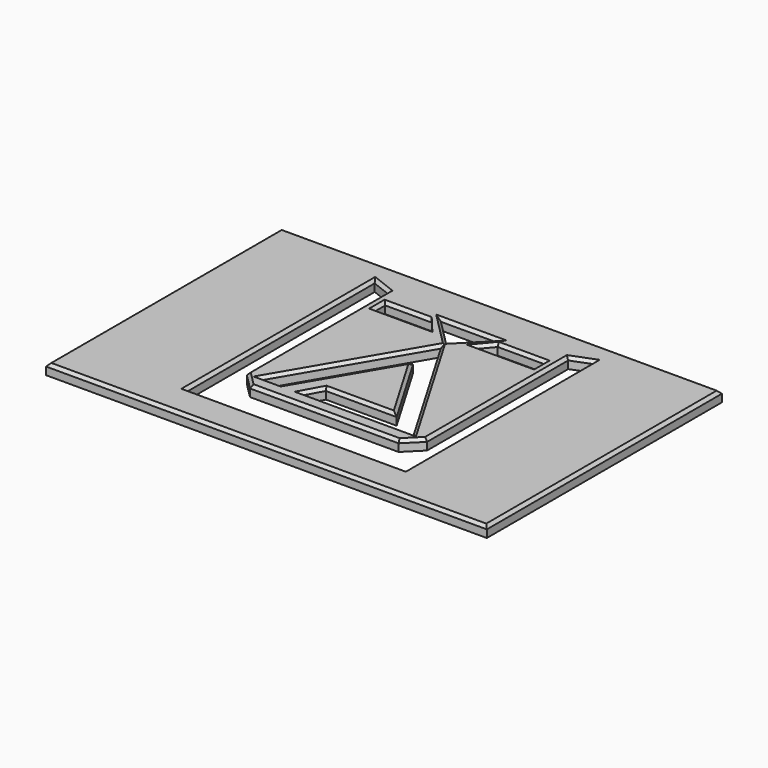
from build123d import *

# Parameters (mm, degrees)
F2_DEPTH      = 0.9
F3_DEPTH      = 5
F4_T1_DEPTH   = 26.285841494
F4_T3_DEPTH   = 38.785841494
F4_T5_DEPTH   = 3.1950298032
F4_T7_DEPTH   = 13.9251834597
F4_T9_DEPTH   = 3.1950298032
F4_T11_DEPTH  = 18.6
F4_T13_DEPTH  = 8.9042054248
F4_T15_DEPTH  = 1.1497265659
F4_T20_DEPTH  = 20.642920747
F4_T25_DEPTH  = 3.035841494
F4_T31_DEPTH  = 16.285841494
F4_T36_DEPTH  = 16.285841494
F4_T41_DEPTH  = 3.035841494
F4_T47_DEPTH  = 20.642920747
F4_T52_DEPTH  = 14.073841494
F4_T58_DEPTH  = 14.073841494
F4_T64_DEPTH  = 10.6487776251
F4_T69_DEPTH  = 7.3005243293
F4_T74_DEPTH  = 3.0018588708
F4_T80_DEPTH  = 10.7389121025
F4_T86_DEPTH  = 3.0133324052
F4_T92_DEPTH  = 5.5681345012
F4_T97_DEPTH  = 4.6046142425
F4_T102_DEPTH = 4.7067640091
F4_T108_DEPTH = 6.1091194569
F4_T114_DEPTH = 4.7067640091
F4_T120_DEPTH = 2.7859223136
F4_T126_DEPTH = 4.6046142425
F4_T131_DEPTH = 5.5681345012
F4_T137_DEPTH = 19.242920747
F4_T141_DEPTH = 21.285841494
F4_T148_DEPTH = 3.035841494
F4_T152_DEPTH = 20.642920747
F4_T159_DEPTH = 16.285841494
F4_T163_DEPTH = 3.035841494
F4_T170_DEPTH = 3.035841494
F4_T174_DEPTH = 16.285841494
F4_T181_DEPTH = 20.642920747
F4_T185_DEPTH = 3.035841494
F4_T192_DEPTH = 19.242920747
F4_T196_DEPTH = 21.285841494
F4_T203_DEPTH = 3.0133324052
F4_T207_DEPTH = 14.073841494
F4_T214_DEPTH = 14.073841494
F4_T218_DEPTH = 14.073841494
F4_T225_DEPTH = 10.7389121025
F4_T229_DEPTH = 14.073841494
F4_T236_DEPTH = 3.0133324052
F4_T240_DEPTH = 10.6487776251
F4_T247_DEPTH = 7.3005243293
F4_T251_DEPTH = 3.0018588708
F4_T258_DEPTH = 3.0018588708
F4_T262_DEPTH = 10.7389121025
F4_T269_DEPTH = 1.7926473129
F4_T273_DEPTH = 6.2110552482
F4_T280_DEPTH = 1.7926473129
F4_T284_DEPTH = 5.2475349895
F4_T291_DEPTH = 4.7067640091
F4_T295_DEPTH = 4.7067640091
F4_T302_DEPTH = 6.1091194569
F4_T306_DEPTH = 4.7067640091
F4_T313_DEPTH = 6.1091194569
F4_T317_DEPTH = 4.7067640091
F4_T324_DEPTH = 2.7859223136
F4_T328_DEPTH = 5.5681345012
F4_T335_DEPTH = 4.6046142425
F4_T339_DEPTH = 2.7859223136
F4_T346_DEPTH = 5.2475349895
F4_T350_DEPTH = 1.7926473129
F4_T357_DEPTH = 6.2110552482
F4_T361_DEPTH = 1.7926473129


# Not quite as in the source:
# - a fillet or chamfer that OpenCascade refuses, or shapes differently, is made with other operations: its cross-section is extruded or revolved along the edge and cut away or added


with BuildPart() as f2:
    # F1 (on Top) → F2 (new body)
    with BuildSketch(Plane.XY):
        Polygon((-18.75, -12), (0, -12), (18.75, -12), (18.75, 13), (-18.75, 13), align=None)
    extrude(amount=F2_DEPTH)

    # F0 (on Top) → F3 (cut)
    with BuildSketch(Plane.XY):
        Polygon((-9.1827595606, 10.9884138033), (-9.1827595606, -9.0115861967), (9.4172404394, -9.0115861967), (9.4172404394, 10.9884138033), (7.7869114222, 10.3523892), (7.7869114222, -4.6476108), (6.4369114222, -5.9976108), (-6.2024305435, -5.9976108), (-7.5524305435, -4.6476108), (-7.5524305435, 10.3523892), align=None)
        Polygon((-2.6888800301, 8.9422948658), (-6.6505735256, 8.9422948658), (-6.6505735256, 7.7925682999), (-1.7253597714, 7.7925682999), align=None)
        Polygon((0.1172404394, 6.394509411), (-6.3555088598, -4.6343826689), (-4.6280179486, -4.6343826689), (0.1170416773, 3.4371092715), (3.9779663485, -3.1304419972), (-2.0367164869, -3.1304419972), (-2.86308087, -4.6343826689), (6.5899897385, -4.6343826689), align=None)
        Polygon((6.8850544043, 8.9422948658), (2.9233609088, 8.9422948658), (1.9598406501, 7.7925682999), (6.8850544043, 7.7925682999), align=None)
        Polygon((2.5288794208, 9.4185657799), (-2.2943985421, 9.4185657799), (0.1172404394, 6.9923118202), align=None)
    extrude(amount=F3_DEPTH, mode=Mode.SUBTRACT)

    # F4: chamfer of 0.25 on 32 edges, made by hand

    # F4_s2 → F4_t1 (cut)
    with BuildSketch(Plane.XZ.offset(-13.642920747)):
        Polygon((-18.75, 0.65), (-18.5, 0.9), (-18.75, 0.9), align=None)
        Polygon((18.5, 0.9), (18.75, 0.65), (18.75, 0.9), align=None)
    extrude(amount=F4_T1_DEPTH, mode=Mode.SUBTRACT)

    # F4_s4 → F4_t3 (cut)
    with BuildSketch(Plane.YZ.offset(-19.392920747)):
        Polygon((12.75, 0.9), (13, 0.65), (13, 0.9), align=None)
        Polygon((-12, 0.65), (-11.75, 0.9), (-12, 0.9), align=None)
    extrude(amount=F4_T3_DEPTH, mode=Mode.SUBTRACT)

    # F4_s6 → F4_t5 (cut)
    with BuildSketch(Plane(origin=(-1.9070234917, 1.9070234917, 0), x_dir=(0, 0, 1), z_dir=(0.7071067812, -0.7071067812, 0))):
        Polygon((0.9, 8.3767319647), (0.65, 8.6267319647), (0.9, 8.6267319647), align=None)
    extrude(amount=F4_T5_DEPTH, mode=Mode.SUBTRACT)

    # F4_s8 → F4_t7 (cut)
    with BuildSketch(Plane.YZ.offset(-6.8453512905)):
        Polygon((-5.7476108, 0.9), (-5.9976108, 0.65), (-5.9976108, 0.9), align=None)
    extrude(amount=F4_T7_DEPTH, mode=Mode.SUBTRACT)

    # F4_s10 → F4_t9 (cut)
    with BuildSketch(Plane(origin=(-0.2349633088, -0.2349633088, 0), x_dir=(0, 0, 1), z_dir=(0.7071067812, 0.7071067812, 0))):
        Polygon((0.9, 8.5425349841), (0.65, 8.7925349841), (0.9, 8.7925349841), align=None)
    extrude(amount=F4_T9_DEPTH, mode=Mode.SUBTRACT)

    # F4_s12 → F4_t11 (cut)
    with BuildSketch(Plane.YZ.offset(-9.1827595606)):
        Polygon((-9.2615861967, 0.9), (-9.0115861967, 0.65), (-9.0115861967, 0.9), align=None)
    extrude(amount=F4_T11_DEPTH, mode=Mode.SUBTRACT)

    # F4_s14 → F4_t13 (cut)
    with BuildSketch(Plane(origin=(2.7151762758, -4.6185981114, 0), x_dir=(0, 0, 1), z_dir=(-0.5067918396, 0.8620684609, 0))):
        Polygon((0.9, 1.5927968692), (0.65, 1.8427968692), (0.9, 1.8427968692), align=None)
    extrude(amount=F4_T13_DEPTH, mode=Mode.SUBTRACT)

    # F4_s16 → F4_t15 (cut)
    with BuildSketch(Plane.XZ.offset(-8.9422948658)):
        Polygon((-6.9005735256, 0.9), (-6.6505735256, 0.65), (-6.6505735256, 0.9), align=None)
        Polygon((7.1350544043, 0.9), (6.8850544043, 0.65), (6.8850544043, 0.9), align=None)
    extrude(amount=F4_T15_DEPTH, mode=Mode.SUBTRACT)


with BuildPart() as f4_tool18:
    # F4_s19 → F4_t20 (new body)
    with BuildSketch(Plane.XZ.offset(9.0115861967)):
        Polygon((-9.4327595606, 0.9), (-9.1827595606, 0.65), (-9.1827595606, 0.9), align=None)
    extrude(amount=-F4_T20_DEPTH)

    split(bisect_by=Plane(origin=(2.5076023076, 6.4277651912, 0), x_dir=(0, 0, 1), z_dir=(-0.3634426304, -0.9316165812, 0)), keep=Keep.TOP)


with BuildPart() as f2_1:
    add(f2.part)

    # F4_t17: cut F4_tool18
    add(f4_tool18.part, mode=Mode.SUBTRACT)


with BuildPart() as f4_tool23:
    # F4_s24 → F4_t25 (new body)
    with BuildSketch(Plane(origin=(-12.2893174966, 4.7943134195, 0), x_dir=(0, 0, 1), z_dir=(0.9316165812, -0.3634426304, 0))):
        Polygon((0.9, -7.149582211), (0.65, -6.899582211), (0.9, -6.899582211), align=None)
    extrude(amount=F4_T25_DEPTH)

    split(bisect_by=Plane.YZ.offset(-7.5524305435), keep=Keep.BOTTOM)

    split(bisect_by=Plane.YZ.offset(-9.1827595606), keep=Keep.TOP)


with BuildPart() as f2_2:
    add(f2_1.part)

    # F4_t22: cut F4_tool23
    add(f4_tool23.part, mode=Mode.SUBTRACT)


with BuildPart() as f4_tool29:
    # F4_s30 → F4_t31 (new body)
    with BuildSketch(Plane.XZ.offset(-10.995309947)):
        Polygon((-7.3024305435, 0.9), (-7.5524305435, 0.65), (-7.5524305435, 0.9), align=None)
    extrude(amount=F4_T31_DEPTH)

    split(bisect_by=Plane(origin=(2.5076023076, 6.4277651912, 0), x_dir=(0, 0, 1), z_dir=(-0.3634426304, -0.9316165812, 0)), keep=Keep.TOP)


with BuildPart() as f2_3:
    add(f2_2.part)

    # F4_t28: cut F4_tool29
    add(f4_tool29.part, mode=Mode.SUBTRACT)


with BuildPart() as f4_tool34:
    # F4_s35 → F4_t36 (new body)
    with BuildSketch(Plane.XZ.offset(5.290531547)):
        Polygon((7.5369114222, 0.9), (7.7869114222, 0.65), (7.7869114222, 0.9), align=None)
    extrude(amount=-F4_T36_DEPTH)

    split(bisect_by=Plane(origin=(-2.4766296004, 6.3483725026, 0), x_dir=(0, 0, 1), z_dir=(0.3634426304, -0.9316165812, 0)), keep=Keep.TOP)


with BuildPart() as f2_4:
    add(f2_3.part)

    # F4_t33: cut F4_tool34
    add(f4_tool34.part, mode=Mode.SUBTRACT)


with BuildPart() as f4_tool39:
    # F4_s40 → F4_t41 (new body)
    with BuildSketch(Plane(origin=(9.6645853944, 3.77035189, 0), x_dir=(0, 0, 1), z_dir=(0.9316165812, 0.3634426304, 0))):
        Polygon((0.9, -7.0643618637), (0.65, -6.8143618637), (0.9, -6.8143618637), align=None)
    extrude(amount=F4_T41_DEPTH)

    split(bisect_by=Plane.YZ.offset(9.4172404394), keep=Keep.BOTTOM)

    split(bisect_by=Plane.YZ.offset(7.7869114222), keep=Keep.TOP)


with BuildPart() as f2_5:
    add(f2_4.part)

    # F4_t38: cut F4_tool39
    add(f4_tool39.part, mode=Mode.SUBTRACT)


with BuildPart() as f4_tool45:
    # F4_s46 → F4_t47 (new body)
    with BuildSketch(Plane.XZ.offset(-11.6313345503)):
        Polygon((9.6672404394, 0.9), (9.4172404394, 0.65), (9.4172404394, 0.9), align=None)
    extrude(amount=F4_T47_DEPTH)

    split(bisect_by=Plane(origin=(-2.4766296004, 6.3483725026, 0), x_dir=(0, 0, 1), z_dir=(0.3634426304, -0.9316165812, 0)), keep=Keep.TOP)


with BuildPart() as f2_6:
    add(f2_5.part)

    # F4_t44: cut F4_tool45
    add(f4_tool45.part, mode=Mode.SUBTRACT)


with BuildPart() as f4_tool50:
    # F4_s51 → F4_t52 (new body)
    with BuildSketch(Plane(origin=(-3.9767285934, -6.7759322138, 0), x_dir=(0, 0, 1), z_dir=(0.5061580622, 0.8624407319, 0))):
        Polygon((0.9, -3.3855195618), (0.65, -3.1355195618), (0.9, -3.1355195618), align=None)
    extrude(amount=F4_T52_DEPTH)

    split(bisect_by=Plane.XZ.offset(4.6343826689), keep=Keep.BOTTOM)

    split(bisect_by=Plane(origin=(2.8786076051, 1.6894267551, 0), x_dir=(0, 0, 1), z_dir=(-0.8624407319, -0.5061580622, 0)), keep=Keep.TOP)


with BuildPart() as f2_7:
    add(f2_6.part)

    # F4_t49: cut F4_tool50
    add(f4_tool50.part, mode=Mode.SUBTRACT)


with BuildPart() as f4_tool56:
    # F4_s57 → F4_t58 (new body)
    with BuildSketch(Plane(origin=(-3.0867866852, 5.2595636956, 0), x_dir=(0, 0, 1), z_dir=(0.5061580622, -0.8624407319, 0))):
        Polygon((0.9, -3.5877454224), (0.65, -3.3377454224), (0.9, -3.3377454224), align=None)
    extrude(amount=F4_T58_DEPTH)

    split(bisect_by=Plane.XZ.offset(4.6343826689), keep=Keep.BOTTOM)

    split(bisect_by=Plane(origin=(-2.7041997858, 1.5870685053, 0), x_dir=(0, 0, 1), z_dir=(0.8624407319, -0.5061580622, 0)), keep=Keep.TOP)


with BuildPart() as f2_8:
    add(f2_7.part)

    # F4_t55: cut F4_tool56
    add(f4_tool56.part, mode=Mode.SUBTRACT)


with BuildPart() as f4_tool62:
    # F4_s63 → F4_t64 (new body)
    with BuildSketch(Plane(origin=(1.8575238649, 3.1597050588, 0), x_dir=(0, 0, 1), z_dir=(-0.5067918396, -0.8620684609, 0))):
        Polygon((0.9, 1.391000992), (0.65, 1.641000992), (0.9, 1.641000992), align=None)
    extrude(amount=F4_T64_DEPTH)

    split(bisect_by=Plane.XZ.offset(4.6343826689), keep=Keep.BOTTOM)


with BuildPart() as f2_9:
    add(f2_8.part)

    # F4_t61: cut F4_tool62
    add(f4_tool62.part, mode=Mode.SUBTRACT)


with BuildPart() as f4_tool67:
    # F4_s68 → F4_t69 (new body)
    with BuildSketch(Plane.YZ.offset(-2.6796372339)):
        Polygon((-2.8804419972, 0.9), (-3.1304419972, 0.65), (-3.1304419972, 0.9), align=None)
    extrude(amount=F4_T69_DEPTH)

    split(bisect_by=Plane(origin=(-0.2432150273, 0.1336384073, 0), x_dir=(0, 0, 1), z_dir=(0.876413428, -0.4815594494, 0)), keep=Keep.TOP)


with BuildPart() as f2_10:
    add(f2_9.part)

    # F4_t66: cut F4_tool67
    add(f4_tool67.part, mode=Mode.SUBTRACT)


with BuildPart() as f4_tool72:
    # F4_s73 → F4_t74 (new body)
    with BuildSketch(Plane(origin=(-2.9294704036, -5.3314854519, 0), x_dir=(0, 0, 1), z_dir=(0.4815594494, 0.876413428, 0))):
        Polygon((0.9, -0.5275117536), (0.65, -0.2775117536), (0.9, -0.2775117536), align=None)
    extrude(amount=F4_T74_DEPTH)

    split(bisect_by=Plane.XZ.offset(3.1304419972), keep=Keep.TOP)

    split(bisect_by=Plane.XZ.offset(4.6343826689), keep=Keep.BOTTOM)


with BuildPart() as f2_11:
    add(f2_10.part)

    # F4_t71: cut F4_tool72
    add(f4_tool72.part, mode=Mode.SUBTRACT)


with BuildPart() as f4_tool78:
    # F4_s79 → F4_t80 (new body)
    with BuildSketch(Plane.YZ.offset(7.2329104855)):
        Polygon((-4.8843826689, 0.9), (-4.6343826689, 0.65), (-4.6343826689, 0.9), align=None)
    extrude(amount=-F4_T80_DEPTH)

    split(bisect_by=Plane(origin=(-0.2432150273, 0.1336384073, 0), x_dir=(0, 0, 1), z_dir=(0.876413428, -0.4815594494, 0)), keep=Keep.TOP)

    split(bisect_by=Plane(origin=(2.8786076051, 1.6894267551, 0), x_dir=(0, 0, 1), z_dir=(-0.8624407319, -0.5061580622, 0)), keep=Keep.TOP)


with BuildPart() as f2_12:
    add(f2_11.part)

    # F4_t77: cut F4_tool78
    add(f4_tool78.part, mode=Mode.SUBTRACT)


with BuildPart() as f4_tool84:
    # F4_s85 → F4_t86 (new body)
    with BuildSketch(Plane.YZ.offset(-3.9850972016)):
        Polygon((-4.8843826689, 0.9), (-4.6343826689, 0.65), (-4.6343826689, 0.9), align=None)
    extrude(amount=-F4_T86_DEPTH)

    split(bisect_by=Plane(origin=(-1.4146551995, 0.8316459115, 0), x_dir=(0, 0, 1), z_dir=(-0.8620684609, 0.5067918396, 0)), keep=Keep.TOP)

    split(bisect_by=Plane(origin=(-2.7041997858, 1.5870685053, 0), x_dir=(0, 0, 1), z_dir=(0.8624407319, -0.5061580622, 0)), keep=Keep.TOP)


with BuildPart() as f2_13:
    add(f2_12.part)

    # F4_t83: cut F4_tool84
    add(f4_tool84.part, mode=Mode.SUBTRACT)


with BuildPart() as f4_tool90:
    # F4_s91 → F4_t92 (new body)
    with BuildSketch(Plane.YZ.offset(-1.0824390244)):
        Polygon((7.5425682999, 0.9), (7.7925682999, 0.65), (7.7925682999, 0.9), align=None)
    extrude(amount=-F4_T92_DEPTH)

    split(bisect_by=Plane(origin=(2.822711668, 2.3655536517, 0), x_dir=(0, 0, 1), z_dir=(-0.7664430815, -0.6423122315, 0)), keep=Keep.TOP)


with BuildPart() as f2_14:
    add(f2_13.part)

    # F4_t89: cut F4_tool90
    add(f4_tool90.part, mode=Mode.SUBTRACT)


with BuildPart() as f4_tool95:
    # F4_s96 → F4_t97 (new body)
    with BuildSketch(Plane.YZ.offset(-6.6505735256)):
        Polygon((9.1922948658, 0.9), (8.9422948658, 0.65), (8.9422948658, 0.9), align=None)
    extrude(amount=F4_T97_DEPTH)

    split(bisect_by=Plane(origin=(2.822711668, 2.3655536517, 0), x_dir=(0, 0, 1), z_dir=(-0.7664430815, -0.6423122315, 0)), keep=Keep.TOP)


with BuildPart() as f2_15:
    add(f2_14.part)

    # F4_t94: cut F4_tool95
    add(f4_tool95.part, mode=Mode.SUBTRACT)


with BuildPart() as f4_tool100:
    # F4_s101 → F4_t102 (new body)
    with BuildSketch(Plane(origin=(-2.9845878597, 3.0026750141, 0), x_dir=(0, 0, 1), z_dir=(-0.7049674381, 0.7092396712, 0))):
        Polygon((0.9, 4.7625037211), (0.65, 5.0125037211), (0.9, 5.0125037211), align=None)
    extrude(amount=F4_T102_DEPTH)

    split(bisect_by=Plane.XZ.offset(-9.4185657799), keep=Keep.TOP)

    split(bisect_by=Plane(origin=(-3.4371177057, 3.4164136073, 0), x_dir=(0, 0, 1), z_dir=(-0.7092396712, 0.7049674381, 0)), keep=Keep.TOP)


with BuildPart() as f2_16:
    add(f2_15.part)

    # F4_t99: cut F4_tool100
    add(f4_tool100.part, mode=Mode.SUBTRACT)


with BuildPart() as f4_tool106:
    # F4_s107 → F4_t108 (new body)
    with BuildSketch(Plane.YZ.offset(-2.9373192891)):
        Polygon((9.6685657799, 0.9), (9.4185657799, 0.65), (9.4185657799, 0.9), align=None)
    extrude(amount=F4_T108_DEPTH)

    split(bisect_by=Plane(origin=(3.555066491, 3.5336519068, 0), x_dir=(0, 0, 1), z_dir=(0.7092396712, 0.7049674381, 0)), keep=Keep.TOP)

    split(bisect_by=Plane(origin=(-3.4371177057, 3.4164136073, 0), x_dir=(0, 0, 1), z_dir=(-0.7092396712, 0.7049674381, 0)), keep=Keep.TOP)


with BuildPart() as f2_17:
    add(f2_16.part)

    # F4_t105: cut F4_tool106
    add(f4_tool106.part, mode=Mode.SUBTRACT)


with BuildPart() as f4_tool112:
    # F4_s113 → F4_t114 (new body)
    with BuildSketch(Plane(origin=(6.4192353184, 6.4581370718, 0), x_dir=(0, 0, 1), z_dir=(-0.7049674381, -0.7092396712, 0))):
        Polygon((0.9, 4.5962005798), (0.65, 4.8462005798), (0.9, 4.8462005798), align=None)
    extrude(amount=F4_T114_DEPTH)

    split(bisect_by=Plane.XZ.offset(-9.4185657799), keep=Keep.TOP)

    split(bisect_by=Plane(origin=(3.555066491, 3.5336519068, 0), x_dir=(0, 0, 1), z_dir=(0.7092396712, 0.7049674381, 0)), keep=Keep.TOP)


with BuildPart() as f2_18:
    add(f2_17.part)

    # F4_t111: cut F4_tool112
    add(f4_tool112.part, mode=Mode.SUBTRACT)


with BuildPart() as f4_tool118:
    # F4_s119 → F4_t120 (new body)
    with BuildSketch(Plane(origin=(4.2318541841, 5.0496864335, 0), x_dir=(0, 0, 1), z_dir=(0.6423122315, 0.7664430815, 0))):
        Polygon((0.9, -3.7531556267), (0.65, -3.5031556267), (0.9, -3.5031556267), align=None)
    extrude(amount=F4_T120_DEPTH)

    split(bisect_by=Plane.XZ.offset(-8.9422948658), keep=Keep.TOP)

    split(bisect_by=Plane.XZ.offset(-7.7925682999), keep=Keep.BOTTOM)


with BuildPart() as f2_19:
    add(f2_18.part)

    # F4_t117: cut F4_tool118
    add(f4_tool118.part, mode=Mode.SUBTRACT)


with BuildPart() as f4_tool124:
    # F4_s125 → F4_t126 (new body)
    with BuildSketch(Plane.YZ.offset(2.2804401618)):
        Polygon((9.1922948658, 0.9), (8.9422948658, 0.65), (8.9422948658, 0.9), align=None)
    extrude(amount=F4_T126_DEPTH)

    split(bisect_by=Plane(origin=(-2.6849693936, 2.2501197079, 0), x_dir=(0, 0, 1), z_dir=(0.7664430815, -0.6423122315, 0)), keep=Keep.TOP)


with BuildPart() as f2_20:
    add(f2_19.part)

    # F4_t123: cut F4_tool124
    add(f4_tool124.part, mode=Mode.SUBTRACT)


with BuildPart() as f4_tool129:
    # F4_s130 → F4_t131 (new body)
    with BuildSketch(Plane.YZ.offset(6.8850544043)):
        Polygon((7.5425682999, 0.9), (7.7925682999, 0.65), (7.7925682999, 0.9), align=None)
    extrude(amount=-F4_T131_DEPTH)

    split(bisect_by=Plane(origin=(-2.6849693936, 2.2501197079, 0), x_dir=(0, 0, 1), z_dir=(0.7664430815, -0.6423122315, 0)), keep=Keep.TOP)


with BuildPart() as f2_21:
    add(f2_20.part)

    # F4_t128: cut F4_tool129
    add(f4_tool129.part, mode=Mode.SUBTRACT)


with BuildPart() as f4_tool135:
    # F4_s136 → F4_t137 (new body)
    with BuildSketch(Plane.YZ.offset(9.4172404394)):
        Polygon((-9.2615861967, 0.9), (-9.0115861967, 0.65), (-9.0115861967, 0.9), align=None)
    extrude(amount=-F4_T137_DEPTH)

    split(bisect_by=Plane.YZ.offset(-9.1827595606), keep=Keep.BOTTOM)


with BuildPart() as f4_tool139:
    # F4_s140 → F4_t141 (new body)
    with BuildSketch(Plane.XZ.offset(9.6545069437)):
        Polygon((-9.4327595606, 0.9), (-9.1827595606, 0.65), (-9.1827595606, 0.9), align=None)
    extrude(amount=-F4_T141_DEPTH)

    split(bisect_by=Plane.XZ.offset(9.0115861967), keep=Keep.TOP)


with BuildPart() as f4_tool135_1:
    add(f4_tool135.part)

    # F4_t143: intersect F4_tool139
    add(f4_tool139.part, mode=Mode.INTERSECT)


with BuildPart() as f2_22:
    add(f2_21.part)

    # F4_t133: cut F4_tool135
    add(f4_tool135_1.part, mode=Mode.SUBTRACT)


with BuildPart() as f4_tool146:
    # F4_s147 → F4_t148 (new body)
    with BuildSketch(Plane(origin=(-12.2893174966, 4.7943134195, 0), x_dir=(0, 0, 1), z_dir=(0.9316165812, -0.3634426304, 0))):
        Polygon((0.9, -7.149582211), (0.65, -6.899582211), (0.9, -6.899582211), align=None)
    extrude(amount=F4_T148_DEPTH)

    split(bisect_by=Plane.YZ.offset(-9.1827595606), keep=Keep.BOTTOM)


with BuildPart() as f4_tool150:
    # F4_s151 → F4_t152 (new body)
    with BuildSketch(Plane.XZ.offset(9.0115861967)):
        Polygon((-9.4327595606, 0.9), (-9.1827595606, 0.65), (-9.1827595606, 0.9), align=None)
    extrude(amount=-F4_T152_DEPTH)

    split(bisect_by=Plane(origin=(2.5076023076, 6.4277651912, 0), x_dir=(0, 0, 1), z_dir=(0.3634426304, 0.9316165812, 0)), keep=Keep.TOP)


with BuildPart() as f4_tool146_1:
    add(f4_tool146.part)

    # F4_t154: intersect F4_tool150
    add(f4_tool150.part, mode=Mode.INTERSECT)


with BuildPart() as f2_23:
    add(f2_22.part)

    # F4_t144: cut F4_tool146
    add(f4_tool146_1.part, mode=Mode.SUBTRACT)


with BuildPart() as f4_tool157:
    # F4_s158 → F4_t159 (new body)
    with BuildSketch(Plane.XZ.offset(-10.995309947)):
        Polygon((-7.3024305435, 0.9), (-7.5524305435, 0.65), (-7.5524305435, 0.9), align=None)
    extrude(amount=F4_T159_DEPTH)

    split(bisect_by=Plane(origin=(2.5076023076, 6.4277651912, 0), x_dir=(0, 0, 1), z_dir=(0.3634426304, 0.9316165812, 0)), keep=Keep.TOP)


with BuildPart() as f4_tool161:
    # F4_s162 → F4_t163 (new body)
    with BuildSketch(Plane(origin=(-12.2893174966, 4.7943134195, 0), x_dir=(0, 0, 1), z_dir=(0.9316165812, -0.3634426304, 0))):
        Polygon((0.9, -7.149582211), (0.65, -6.899582211), (0.9, -6.899582211), align=None)
    extrude(amount=F4_T163_DEPTH)

    split(bisect_by=Plane.YZ.offset(-7.5524305435), keep=Keep.TOP)


with BuildPart() as f4_tool157_1:
    add(f4_tool157.part)

    # F4_t165: intersect F4_tool161
    add(f4_tool161.part, mode=Mode.INTERSECT)


with BuildPart() as f2_24:
    add(f2_23.part)

    # F4_t155: cut F4_tool157
    add(f4_tool157_1.part, mode=Mode.SUBTRACT)


with BuildPart() as f4_tool168:
    # F4_s169 → F4_t170 (new body)
    with BuildSketch(Plane(origin=(9.6645853944, 3.77035189, 0), x_dir=(0, 0, 1), z_dir=(0.9316165812, 0.3634426304, 0))):
        Polygon((0.9, -7.0643618637), (0.65, -6.8143618637), (0.9, -6.8143618637), align=None)
    extrude(amount=F4_T170_DEPTH)

    split(bisect_by=Plane.YZ.offset(7.7869114222), keep=Keep.BOTTOM)


with BuildPart() as f4_tool172:
    # F4_s173 → F4_t174 (new body)
    with BuildSketch(Plane.XZ.offset(5.290531547)):
        Polygon((7.5369114222, 0.9), (7.7869114222, 0.65), (7.7869114222, 0.9), align=None)
    extrude(amount=-F4_T174_DEPTH)

    split(bisect_by=Plane(origin=(-2.4766296004, 6.3483725026, 0), x_dir=(0, 0, 1), z_dir=(-0.3634426304, 0.9316165812, 0)), keep=Keep.TOP)


with BuildPart() as f4_tool168_1:
    add(f4_tool168.part)

    # F4_t176: intersect F4_tool172
    add(f4_tool172.part, mode=Mode.INTERSECT)


with BuildPart() as f2_25:
    add(f2_24.part)

    # F4_t166: cut F4_tool168
    add(f4_tool168_1.part, mode=Mode.SUBTRACT)


with BuildPart() as f4_tool179:
    # F4_s180 → F4_t181 (new body)
    with BuildSketch(Plane.XZ.offset(-11.6313345503)):
        Polygon((9.6672404394, 0.9), (9.4172404394, 0.65), (9.4172404394, 0.9), align=None)
    extrude(amount=F4_T181_DEPTH)

    split(bisect_by=Plane(origin=(-2.4766296004, 6.3483725026, 0), x_dir=(0, 0, 1), z_dir=(-0.3634426304, 0.9316165812, 0)), keep=Keep.TOP)


with BuildPart() as f4_tool183:
    # F4_s184 → F4_t185 (new body)
    with BuildSketch(Plane(origin=(9.6645853944, 3.77035189, 0), x_dir=(0, 0, 1), z_dir=(0.9316165812, 0.3634426304, 0))):
        Polygon((0.9, -7.0643618637), (0.65, -6.8143618637), (0.9, -6.8143618637), align=None)
    extrude(amount=F4_T185_DEPTH)

    split(bisect_by=Plane.YZ.offset(9.4172404394), keep=Keep.TOP)


with BuildPart() as f4_tool179_1:
    add(f4_tool179.part)

    # F4_t187: intersect F4_tool183
    add(f4_tool183.part, mode=Mode.INTERSECT)


with BuildPart() as f2_26:
    add(f2_25.part)

    # F4_t177: cut F4_tool179
    add(f4_tool179_1.part, mode=Mode.SUBTRACT)


with BuildPart() as f4_tool190:
    # F4_s191 → F4_t192 (new body)
    with BuildSketch(Plane.YZ.offset(10.0601611863)):
        Polygon((-9.2615861967, 0.9), (-9.0115861967, 0.65), (-9.0115861967, 0.9), align=None)
    extrude(amount=-F4_T192_DEPTH)

    split(bisect_by=Plane.YZ.offset(9.4172404394), keep=Keep.TOP)


with BuildPart() as f4_tool194:
    # F4_s195 → F4_t196 (new body)
    with BuildSketch(Plane.XZ.offset(-11.6313345503)):
        Polygon((9.6672404394, 0.9), (9.4172404394, 0.65), (9.4172404394, 0.9), align=None)
    extrude(amount=F4_T196_DEPTH)

    split(bisect_by=Plane.XZ.offset(9.0115861967), keep=Keep.TOP)


with BuildPart() as f4_tool190_1:
    add(f4_tool190.part)

    # F4_t198: intersect F4_tool194
    add(f4_tool194.part, mode=Mode.INTERSECT)


with BuildPart() as f2_27:
    add(f2_26.part)

    # F4_t188: cut F4_tool190
    add(f4_tool190_1.part, mode=Mode.SUBTRACT)


with BuildPart() as f4_tool201:
    # F4_s202 → F4_t203 (new body)
    with BuildSketch(Plane.YZ.offset(-3.9850972016)):
        Polygon((-4.8843826689, 0.9), (-4.6343826689, 0.65), (-4.6343826689, 0.9), align=None)
    extrude(amount=-F4_T203_DEPTH)

    split(bisect_by=Plane(origin=(-2.7041997858, 1.5870685053, 0), x_dir=(0, 0, 1), z_dir=(-0.8624407319, 0.5061580622, 0)), keep=Keep.TOP)


with BuildPart() as f4_tool205:
    # F4_s206 → F4_t207 (new body)
    with BuildSketch(Plane(origin=(-3.9767285934, -6.7759322138, 0), x_dir=(0, 0, 1), z_dir=(0.5061580622, 0.8624407319, 0))):
        Polygon((0.9, -3.3855195618), (0.65, -3.1355195618), (0.9, -3.1355195618), align=None)
    extrude(amount=F4_T207_DEPTH)

    split(bisect_by=Plane.XZ.offset(4.6343826689), keep=Keep.TOP)


with BuildPart() as f4_tool201_1:
    add(f4_tool201.part)

    # F4_t209: intersect F4_tool205
    add(f4_tool205.part, mode=Mode.INTERSECT)


with BuildPart() as f2_28:
    add(f2_27.part)

    # F4_t199: cut F4_tool201
    add(f4_tool201_1.part, mode=Mode.SUBTRACT)


with BuildPart() as f4_tool212:
    # F4_s213 → F4_t214 (new body)
    with BuildSketch(Plane(origin=(-3.0867866852, 5.2595636956, 0), x_dir=(0, 0, 1), z_dir=(0.5061580622, -0.8624407319, 0))):
        Polygon((0.9, -3.5877454224), (0.65, -3.3377454224), (0.9, -3.3377454224), align=None)
    extrude(amount=F4_T214_DEPTH)

    split(bisect_by=Plane(origin=(-2.7041997858, 1.5870685053, 0), x_dir=(0, 0, 1), z_dir=(-0.8624407319, 0.5061580622, 0)), keep=Keep.TOP)


with BuildPart() as f4_tool216:
    # F4_s217 → F4_t218 (new body)
    with BuildSketch(Plane(origin=(-3.9767285934, -6.7759322138, 0), x_dir=(0, 0, 1), z_dir=(0.5061580622, 0.8624407319, 0))):
        Polygon((0.9, -3.3855195618), (0.65, -3.1355195618), (0.9, -3.1355195618), align=None)
    extrude(amount=F4_T218_DEPTH)

    split(bisect_by=Plane(origin=(2.8786076051, 1.6894267551, 0), x_dir=(0, 0, 1), z_dir=(0.8624407319, 0.5061580622, 0)), keep=Keep.TOP)


with BuildPart() as f4_tool212_1:
    add(f4_tool212.part)

    # F4_t220: intersect F4_tool216
    add(f4_tool216.part, mode=Mode.INTERSECT)


with BuildPart() as f2_29:
    add(f2_28.part)

    # F4_t210: cut F4_tool212
    add(f4_tool212_1.part, mode=Mode.SUBTRACT)


with BuildPart() as f4_tool223:
    # F4_s224 → F4_t225 (new body)
    with BuildSketch(Plane.YZ.offset(7.2329104855)):
        Polygon((-4.8843826689, 0.9), (-4.6343826689, 0.65), (-4.6343826689, 0.9), align=None)
    extrude(amount=-F4_T225_DEPTH)

    split(bisect_by=Plane(origin=(2.8786076051, 1.6894267551, 0), x_dir=(0, 0, 1), z_dir=(0.8624407319, 0.5061580622, 0)), keep=Keep.TOP)


with BuildPart() as f4_tool227:
    # F4_s228 → F4_t229 (new body)
    with BuildSketch(Plane(origin=(-3.0867866852, 5.2595636956, 0), x_dir=(0, 0, 1), z_dir=(0.5061580622, -0.8624407319, 0))):
        Polygon((0.9, -3.5877454224), (0.65, -3.3377454224), (0.9, -3.3377454224), align=None)
    extrude(amount=F4_T229_DEPTH)

    split(bisect_by=Plane.XZ.offset(4.6343826689), keep=Keep.TOP)


with BuildPart() as f4_tool223_1:
    add(f4_tool223.part)

    # F4_t231: intersect F4_tool227
    add(f4_tool227.part, mode=Mode.INTERSECT)


with BuildPart() as f2_30:
    add(f2_29.part)

    # F4_t221: cut F4_tool223
    add(f4_tool223_1.part, mode=Mode.SUBTRACT)


with BuildPart() as f4_tool234:
    # F4_s235 → F4_t236 (new body)
    with BuildSketch(Plane.YZ.offset(-3.9850972016)):
        Polygon((-4.8843826689, 0.9), (-4.6343826689, 0.65), (-4.6343826689, 0.9), align=None)
    extrude(amount=-F4_T236_DEPTH)

    split(bisect_by=Plane(origin=(-1.4146551995, 0.8316459115, 0), x_dir=(0, 0, 1), z_dir=(0.8620684609, -0.5067918396, 0)), keep=Keep.TOP)


with BuildPart() as f4_tool238:
    # F4_s239 → F4_t240 (new body)
    with BuildSketch(Plane(origin=(1.8575238649, 3.1597050588, 0), x_dir=(0, 0, 1), z_dir=(-0.5067918396, -0.8620684609, 0))):
        Polygon((0.9, 1.391000992), (0.65, 1.641000992), (0.9, 1.641000992), align=None)
    extrude(amount=F4_T240_DEPTH)

    split(bisect_by=Plane.XZ.offset(4.6343826689), keep=Keep.TOP)


with BuildPart() as f4_tool234_1:
    add(f4_tool234.part)

    # F4_t242: intersect F4_tool238
    add(f4_tool238.part, mode=Mode.INTERSECT)


with BuildPart() as f2_31:
    add(f2_30.part)

    # F4_t232: cut F4_tool234
    add(f4_tool234_1.part, mode=Mode.SUBTRACT)


with BuildPart() as f4_tool245:
    # F4_s246 → F4_t247 (new body)
    with BuildSketch(Plane.YZ.offset(-2.6796372339)):
        Polygon((-2.8804419972, 0.9), (-3.1304419972, 0.65), (-3.1304419972, 0.9), align=None)
    extrude(amount=F4_T247_DEPTH)

    split(bisect_by=Plane(origin=(-0.2432150273, 0.1336384073, 0), x_dir=(0, 0, 1), z_dir=(-0.876413428, 0.4815594494, 0)), keep=Keep.TOP)


with BuildPart() as f4_tool249:
    # F4_s250 → F4_t251 (new body)
    with BuildSketch(Plane(origin=(-2.9294704036, -5.3314854519, 0), x_dir=(0, 0, 1), z_dir=(0.4815594494, 0.876413428, 0))):
        Polygon((0.9, -0.5275117536), (0.65, -0.2775117536), (0.9, -0.2775117536), align=None)
    extrude(amount=F4_T251_DEPTH)

    split(bisect_by=Plane.XZ.offset(3.1304419972), keep=Keep.BOTTOM)


with BuildPart() as f4_tool245_1:
    add(f4_tool245.part)

    # F4_t253: intersect F4_tool249
    add(f4_tool249.part, mode=Mode.INTERSECT)


with BuildPart() as f2_32:
    add(f2_31.part)

    # F4_t243: cut F4_tool245
    add(f4_tool245_1.part, mode=Mode.SUBTRACT)


with BuildPart() as f4_tool256:
    # F4_s257 → F4_t258 (new body)
    with BuildSketch(Plane(origin=(-2.9294704036, -5.3314854519, 0), x_dir=(0, 0, 1), z_dir=(0.4815594494, 0.876413428, 0))):
        Polygon((0.9, -0.5275117536), (0.65, -0.2775117536), (0.9, -0.2775117536), align=None)
    extrude(amount=F4_T258_DEPTH)

    split(bisect_by=Plane.XZ.offset(4.6343826689), keep=Keep.TOP)


with BuildPart() as f4_tool260:
    # F4_s261 → F4_t262 (new body)
    with BuildSketch(Plane.YZ.offset(7.2329104855)):
        Polygon((-4.8843826689, 0.9), (-4.6343826689, 0.65), (-4.6343826689, 0.9), align=None)
    extrude(amount=-F4_T262_DEPTH)

    split(bisect_by=Plane(origin=(-0.2432150273, 0.1336384073, 0), x_dir=(0, 0, 1), z_dir=(-0.876413428, 0.4815594494, 0)), keep=Keep.TOP)


with BuildPart() as f4_tool256_1:
    add(f4_tool256.part)

    # F4_t264: intersect F4_tool260
    add(f4_tool260.part, mode=Mode.INTERSECT)


with BuildPart() as f2_33:
    add(f2_32.part)

    # F4_t254: cut F4_tool256
    add(f4_tool256_1.part, mode=Mode.SUBTRACT)


with BuildPart() as f4_tool267:
    # F4_s268 → F4_t269 (new body)
    with BuildSketch(Plane.XZ.offset(-7.1496475529)):
        Polygon((-6.9005735256, 0.9), (-6.6505735256, 0.65), (-6.6505735256, 0.9), align=None)
    extrude(amount=-F4_T269_DEPTH)

    split(bisect_by=Plane.XZ.offset(-7.7925682999), keep=Keep.TOP)


with BuildPart() as f4_tool271:
    # F4_s272 → F4_t273 (new body)
    with BuildSketch(Plane.YZ.offset(-1.0824390244)):
        Polygon((7.5425682999, 0.9), (7.7925682999, 0.65), (7.7925682999, 0.9), align=None)
    extrude(amount=-F4_T273_DEPTH)

    split(bisect_by=Plane.YZ.offset(-6.6505735256), keep=Keep.BOTTOM)


with BuildPart() as f4_tool267_1:
    add(f4_tool267.part)

    # F4_t275: intersect F4_tool271
    add(f4_tool271.part, mode=Mode.INTERSECT)


with BuildPart() as f2_34:
    add(f2_33.part)

    # F4_t265: cut F4_tool267
    add(f4_tool267_1.part, mode=Mode.SUBTRACT)


with BuildPart() as f4_tool278:
    # F4_s279 → F4_t280 (new body)
    with BuildSketch(Plane.XZ.offset(-7.7925682999)):
        Polygon((-6.9005735256, 0.9), (-6.6505735256, 0.65), (-6.6505735256, 0.9), align=None)
    extrude(amount=-F4_T280_DEPTH)

    split(bisect_by=Plane.XZ.offset(-8.9422948658), keep=Keep.BOTTOM)


with BuildPart() as f4_tool282:
    # F4_s283 → F4_t284 (new body)
    with BuildSketch(Plane.YZ.offset(-7.2934942726)):
        Polygon((9.1922948658, 0.9), (8.9422948658, 0.65), (8.9422948658, 0.9), align=None)
    extrude(amount=F4_T284_DEPTH)

    split(bisect_by=Plane.YZ.offset(-6.6505735256), keep=Keep.BOTTOM)


with BuildPart() as f4_tool278_1:
    add(f4_tool278.part)

    # F4_t286: intersect F4_tool282
    add(f4_tool282.part, mode=Mode.INTERSECT)


with BuildPart() as f2_35:
    add(f2_34.part)

    # F4_t276: cut F4_tool278
    add(f4_tool278_1.part, mode=Mode.SUBTRACT)


with BuildPart() as f4_tool289:
    # F4_s290 → F4_t291 (new body)
    with BuildSketch(Plane(origin=(-2.9845878597, 3.0026750141, 0), x_dir=(0, 0, 1), z_dir=(-0.7049674381, 0.7092396712, 0))):
        Polygon((0.9, 4.7625037211), (0.65, 5.0125037211), (0.9, 5.0125037211), align=None)
    extrude(amount=F4_T291_DEPTH)

    split(bisect_by=Plane(origin=(-3.4371177057, 3.4164136073, 0), x_dir=(0, 0, 1), z_dir=(0.7092396712, -0.7049674381, 0)), keep=Keep.TOP)


with BuildPart() as f4_tool293:
    # F4_s294 → F4_t295 (new body)
    with BuildSketch(Plane(origin=(6.4192353184, 6.4581370718, 0), x_dir=(0, 0, 1), z_dir=(-0.7049674381, -0.7092396712, 0))):
        Polygon((0.9, 4.5962005798), (0.65, 4.8462005798), (0.9, 4.8462005798), align=None)
    extrude(amount=F4_T295_DEPTH)

    split(bisect_by=Plane(origin=(3.555066491, 3.5336519068, 0), x_dir=(0, 0, 1), z_dir=(-0.7092396712, -0.7049674381, 0)), keep=Keep.TOP)


with BuildPart() as f4_tool289_1:
    add(f4_tool289.part)

    # F4_t297: intersect F4_tool293
    add(f4_tool293.part, mode=Mode.INTERSECT)


with BuildPart() as f2_36:
    add(f2_35.part)

    # F4_t287: cut F4_tool289
    add(f4_tool289_1.part, mode=Mode.SUBTRACT)


with BuildPart() as f4_tool300:
    # F4_s301 → F4_t302 (new body)
    with BuildSketch(Plane.YZ.offset(-2.9373192891)):
        Polygon((9.6685657799, 0.9), (9.4185657799, 0.65), (9.4185657799, 0.9), align=None)
    extrude(amount=F4_T302_DEPTH)

    split(bisect_by=Plane(origin=(3.555066491, 3.5336519068, 0), x_dir=(0, 0, 1), z_dir=(-0.7092396712, -0.7049674381, 0)), keep=Keep.TOP)


with BuildPart() as f4_tool304:
    # F4_s305 → F4_t306 (new body)
    with BuildSketch(Plane(origin=(-2.9845878597, 3.0026750141, 0), x_dir=(0, 0, 1), z_dir=(-0.7049674381, 0.7092396712, 0))):
        Polygon((0.9, 4.7625037211), (0.65, 5.0125037211), (0.9, 5.0125037211), align=None)
    extrude(amount=F4_T306_DEPTH)

    split(bisect_by=Plane.XZ.offset(-9.4185657799), keep=Keep.BOTTOM)


with BuildPart() as f4_tool300_1:
    add(f4_tool300.part)

    # F4_t308: intersect F4_tool304
    add(f4_tool304.part, mode=Mode.INTERSECT)


with BuildPart() as f2_37:
    add(f2_36.part)

    # F4_t298: cut F4_tool300
    add(f4_tool300_1.part, mode=Mode.SUBTRACT)


with BuildPart() as f4_tool311:
    # F4_s312 → F4_t313 (new body)
    with BuildSketch(Plane.YZ.offset(-2.9373192891)):
        Polygon((9.6685657799, 0.9), (9.4185657799, 0.65), (9.4185657799, 0.9), align=None)
    extrude(amount=F4_T313_DEPTH)

    split(bisect_by=Plane(origin=(-3.4371177057, 3.4164136073, 0), x_dir=(0, 0, 1), z_dir=(0.7092396712, -0.7049674381, 0)), keep=Keep.TOP)


with BuildPart() as f4_tool315:
    # F4_s316 → F4_t317 (new body)
    with BuildSketch(Plane(origin=(6.4192353184, 6.4581370718, 0), x_dir=(0, 0, 1), z_dir=(-0.7049674381, -0.7092396712, 0))):
        Polygon((0.9, 4.5962005798), (0.65, 4.8462005798), (0.9, 4.8462005798), align=None)
    extrude(amount=F4_T317_DEPTH)

    split(bisect_by=Plane.XZ.offset(-9.4185657799), keep=Keep.BOTTOM)


with BuildPart() as f4_tool311_1:
    add(f4_tool311.part)

    # F4_t319: intersect F4_tool315
    add(f4_tool315.part, mode=Mode.INTERSECT)


with BuildPart() as f2_38:
    add(f2_37.part)

    # F4_t309: cut F4_tool311
    add(f4_tool311_1.part, mode=Mode.SUBTRACT)


with BuildPart() as f4_tool322:
    # F4_s323 → F4_t324 (new body)
    with BuildSketch(Plane(origin=(4.2318541841, 5.0496864335, 0), x_dir=(0, 0, 1), z_dir=(0.6423122315, 0.7664430815, 0))):
        Polygon((0.9, -3.7531556267), (0.65, -3.5031556267), (0.9, -3.5031556267), align=None)
    extrude(amount=F4_T324_DEPTH)

    split(bisect_by=Plane.XZ.offset(-7.7925682999), keep=Keep.TOP)


with BuildPart() as f4_tool326:
    # F4_s327 → F4_t328 (new body)
    with BuildSketch(Plane.YZ.offset(6.8850544043)):
        Polygon((7.5425682999, 0.9), (7.7925682999, 0.65), (7.7925682999, 0.9), align=None)
    extrude(amount=-F4_T328_DEPTH)

    split(bisect_by=Plane(origin=(-2.6849693936, 2.2501197079, 0), x_dir=(0, 0, 1), z_dir=(-0.7664430815, 0.6423122315, 0)), keep=Keep.TOP)


with BuildPart() as f4_tool322_1:
    add(f4_tool322.part)

    # F4_t330: intersect F4_tool326
    add(f4_tool326.part, mode=Mode.INTERSECT)


with BuildPart() as f2_39:
    add(f2_38.part)

    # F4_t320: cut F4_tool322
    add(f4_tool322_1.part, mode=Mode.SUBTRACT)


with BuildPart() as f4_tool333:
    # F4_s334 → F4_t335 (new body)
    with BuildSketch(Plane.YZ.offset(2.2804401618)):
        Polygon((9.1922948658, 0.9), (8.9422948658, 0.65), (8.9422948658, 0.9), align=None)
    extrude(amount=F4_T335_DEPTH)

    split(bisect_by=Plane(origin=(-2.6849693936, 2.2501197079, 0), x_dir=(0, 0, 1), z_dir=(-0.7664430815, 0.6423122315, 0)), keep=Keep.TOP)


with BuildPart() as f4_tool337:
    # F4_s338 → F4_t339 (new body)
    with BuildSketch(Plane(origin=(4.2318541841, 5.0496864335, 0), x_dir=(0, 0, 1), z_dir=(0.6423122315, 0.7664430815, 0))):
        Polygon((0.9, -3.7531556267), (0.65, -3.5031556267), (0.9, -3.5031556267), align=None)
    extrude(amount=F4_T339_DEPTH)

    split(bisect_by=Plane.XZ.offset(-8.9422948658), keep=Keep.BOTTOM)


with BuildPart() as f4_tool333_1:
    add(f4_tool333.part)

    # F4_t341: intersect F4_tool337
    add(f4_tool337.part, mode=Mode.INTERSECT)


with BuildPart() as f2_40:
    add(f2_39.part)

    # F4_t331: cut F4_tool333
    add(f4_tool333_1.part, mode=Mode.SUBTRACT)


with BuildPart() as f4_tool344:
    # F4_s345 → F4_t346 (new body)
    with BuildSketch(Plane.YZ.offset(2.2804401618)):
        Polygon((9.1922948658, 0.9), (8.9422948658, 0.65), (8.9422948658, 0.9), align=None)
    extrude(amount=F4_T346_DEPTH)

    split(bisect_by=Plane.YZ.offset(6.8850544043), keep=Keep.TOP)


with BuildPart() as f4_tool348:
    # F4_s349 → F4_t350 (new body)
    with BuildSketch(Plane.XZ.offset(-9.5852156128)):
        Polygon((7.1350544043, 0.9), (6.8850544043, 0.65), (6.8850544043, 0.9), align=None)
    extrude(amount=F4_T350_DEPTH)

    split(bisect_by=Plane.XZ.offset(-8.9422948658), keep=Keep.BOTTOM)


with BuildPart() as f4_tool344_1:
    add(f4_tool344.part)

    # F4_t352: intersect F4_tool348
    add(f4_tool348.part, mode=Mode.INTERSECT)


with BuildPart() as f2_41:
    add(f2_40.part)

    # F4_t342: cut F4_tool344
    add(f4_tool344_1.part, mode=Mode.SUBTRACT)


with BuildPart() as f4_tool355:
    # F4_s356 → F4_t357 (new body)
    with BuildSketch(Plane.YZ.offset(7.5279751513)):
        Polygon((7.5425682999, 0.9), (7.7925682999, 0.65), (7.7925682999, 0.9), align=None)
    extrude(amount=-F4_T357_DEPTH)

    split(bisect_by=Plane.YZ.offset(6.8850544043), keep=Keep.TOP)


with BuildPart() as f4_tool359:
    # F4_s360 → F4_t361 (new body)
    with BuildSketch(Plane.XZ.offset(-8.9422948658)):
        Polygon((7.1350544043, 0.9), (6.8850544043, 0.65), (6.8850544043, 0.9), align=None)
    extrude(amount=F4_T361_DEPTH)

    split(bisect_by=Plane.XZ.offset(-7.7925682999), keep=Keep.TOP)


with BuildPart() as f4_tool355_1:
    add(f4_tool355.part)

    # F4_t363: intersect F4_tool359
    add(f4_tool359.part, mode=Mode.INTERSECT)


with BuildPart() as f2_42:
    add(f2_41.part)

    # F4_t353: cut F4_tool355
    add(f4_tool355_1.part, mode=Mode.SUBTRACT)


solid = f2_42.part
